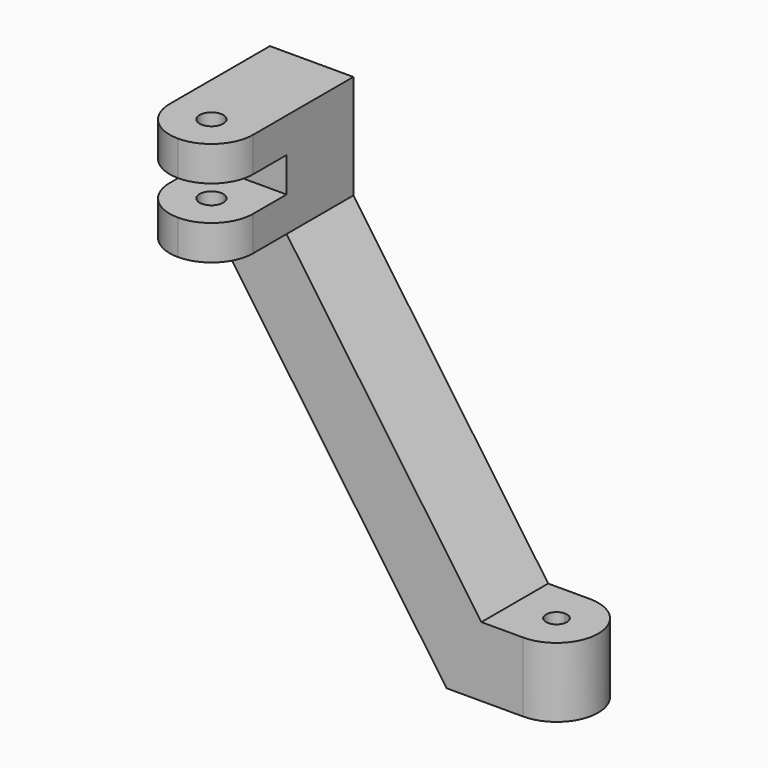
from build123d import *

# Parameters (mm, degrees)
F1_DEPTH  = 20
F2_START  = 10
F1_FACE_R = 1.5
F2_DEPTH  = 10
F3_DEPTH  = 50
F5_DEPTH  = 12.001
F6_DEPTH  = 15
F7_W      = 12
F7_H      = 5
F8_DEPTH  = 12
F9_R      = 5.99999
F11_D     = 3.4


# Not quite as in the source:
# - a fillet or chamfer is up to 0.001 mm smaller than in the source, because OpenCascade refuses the exact size
# - a feature names something its author has since deleted; it is built from what else it names


with BuildPart() as f1:
    # F0 (on Top) → F1 (new body)
    with BuildSketch(Plane.XY):
        with BuildLine():
            ThreePointArc((16, -2), (22, 4), (16, 10))
            Line((16, 10), (16, 5.5))
            ThreePointArc((16, 5.5), (17.0606601718, 5.0606601718), (17.5, 4))
            ThreePointArc((17.5, 4), (17.0606601718, 2.9393398282), (16, 2.5))
            Line((16, 2.5), (16, -2))
        make_face()
        with BuildLine():
            Line((16, 5.5), (16, 10))
            ThreePointArc((16, 10), (11.7573593129, 8.2426406871), (10, 4))
            ThreePointArc((10, 4), (11.7573593129, -0.2426406871), (16, -2))
            Line((16, -2), (16, 2.5))
            ThreePointArc((16, 2.5), (14.5, 4), (16, 5.5))
        make_face()
        with BuildLine():
            Line((16, 10), (10, 10))
            Line((10, 10), (10, 4))
            ThreePointArc((10, 4), (11.7573593129, 8.2426406871), (16, 10))
        make_face()
        with BuildLine():
            ThreePointArc((16, -2), (11.7573593129, -0.2426406871), (10, 4))
            Line((10, 4), (10, -2))
            Line((10, -2), (16, -2))
        make_face()
    extrude(amount=F1_DEPTH)

    # F0 (on Top) + F1_face (on face) → F2 (cut)
    with BuildSketch(Plane.XY.offset(F2_START)):
        with BuildLine():
            ThreePointArc((16, -2), (22, 4), (16, 10))
            Line((16, 10), (16, 5.5))
            ThreePointArc((16, 5.5), (17.0606601718, 5.0606601718), (17.5, 4))
            ThreePointArc((17.5, 4), (17.0606601718, 2.9393398282), (16, 2.5))
            Line((16, 2.5), (16, -2))
        make_face()
        with BuildLine():
            Line((16, 5.5), (16, 10))
            ThreePointArc((16, 10), (11.7573593129, 8.2426406871), (10, 4))
            ThreePointArc((10, 4), (11.7573593129, -0.2426406871), (16, -2))
            Line((16, -2), (16, 2.5))
            ThreePointArc((16, 2.5), (14.5, 4), (16, 5.5))
        make_face()
        with BuildLine():
            ThreePointArc((16, -2), (11.7573593129, -0.2426406871), (10, 4))
            Line((10, 4), (10, -2))
            Line((10, -2), (16, -2))
        make_face()
        with BuildLine():
            Line((16, 10), (10, 10))
            Line((10, 10), (10, 4))
            ThreePointArc((10, 4), (11.7573593129, 8.2426406871), (16, 10))
        make_face()
    with BuildSketch(Plane(origin=(15.4073102565, 4, 20), x_dir=(1, 0, 0), z_dir=(0, 0, 1)).offset(F2_START)):
        with BuildLine():
            ThreePointArc((0.5926897435, -6), (6.5926897435, 0), (0.5926897435, 6))
            Line((0.5926897435, 6), (-5.4073102565, 6))
            Line((-5.4073102565, 6), (-5.4073102565, -6))
            Line((-5.4073102565, -6), (0.5926897435, -6))
        make_face()
        with Locations((0.5926897435, 0)):
            Circle(F1_FACE_R, mode=Mode.SUBTRACT)
    extrude(amount=F2_DEPTH, mode=Mode.SUBTRACT)

    # F0 (on Top) → F3 (join)
    with BuildSketch(Plane.XY):
        Polygon((10, 4), (10, 10), (-30, 10), (-30, -2), (10, -2), align=None)
    extrude(amount=F3_DEPTH)

    # F4 (on face) → F5 (cut, through all)
    with BuildSketch(Plane(origin=(0, 10, 0), x_dir=(-1, 0, 0), z_dir=(0, 1, 0))):
        Polygon((-10, 50), (-10, 10), (18, 50), align=None)
        Polygon((30, 0), (30, 50), (-5, 0), align=None)
    extrude(amount=-F5_DEPTH, mode=Mode.SUBTRACT)

    # F6 (add): a face of the model
    f6_faces = [f1.faces().sort_by_distance(p)[0] for p in [
        (-24, 4, 50),
    ]]
    extrude(f6_faces, amount=F6_DEPTH)

    # F7 (on face) → F8 (join)
    with BuildSketch(Plane.XZ.offset(2)):
        with Locations((-24, 52.5)):
            Rectangle(F7_W, F7_H)
        with Locations((-24, 62.5)):
            Rectangle(F7_W, F7_H)
    extrude(amount=F8_DEPTH)

    # F9 (radius 6 in the source; OpenCascade refuses exactly that, so slightly less here)
    f9_edges = [f1.edges().sort_by_distance(p)[0] for p in [
        (-30, -14, 62.5),
        (-18, -14, 62.5),
        (-18, -14, 52.5),
        (-30, -14, 52.5),
    ]]
    fillet(f9_edges, radius=F9_R)

    # F11 (through all)
    with Locations(Plane.XY.offset(65)):
        with Locations((-24, -8)):
            Hole(F11_D / 2)


solid = f1.part
